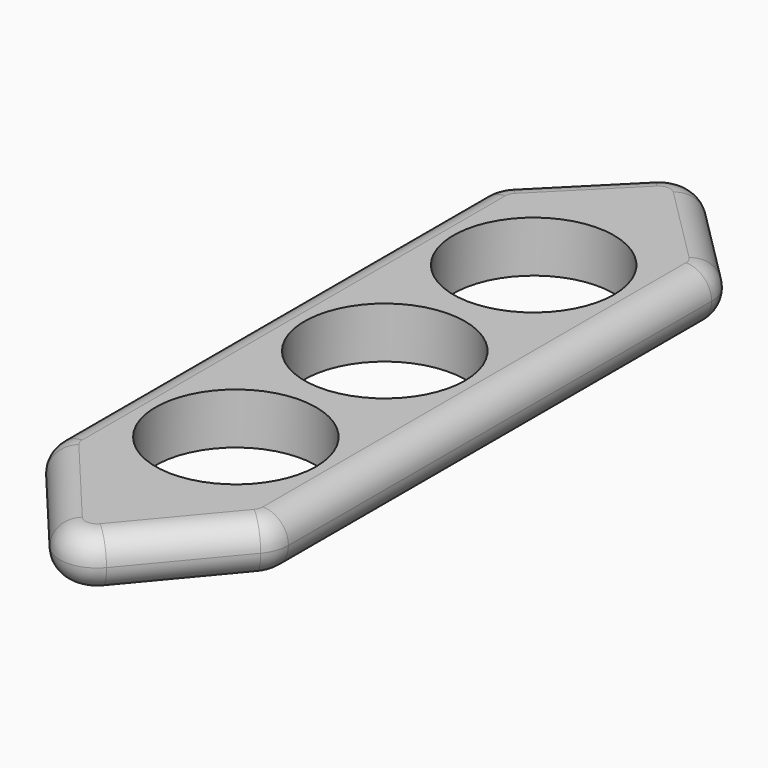
from build123d import *

# Parameters (mm, degrees)
F1_R     = 10.99185
F2_DEPTH = 7
F3_R     = 5.08
F4_R     = 3.49999


# Not quite as in the source:
# - a fillet or chamfer is up to 0.001 mm smaller than in the source, because OpenCascade refuses the exact size


with BuildPart() as f2:
    # F1 (on Top) → F2 (new body)
    with BuildSketch(Plane.XY):
        Polygon((0, 54.0587), (-15.875, 38.1837), (-15.875, -38.1837), (0, -57.15), (15.875, -38.1837), (15.875, 38.1837), align=None)
        with Locations((0, -25.4837)):
            Circle(F1_R, mode=Mode.SUBTRACT)
        Circle(F1_R, mode=Mode.SUBTRACT)
        with Locations((0, 25.4837)):
            Circle(F1_R, mode=Mode.SUBTRACT)
    extrude(amount=F2_DEPTH)

    # F3
    f3_edges = [f2.edges().sort_by_distance(p)[0] for p in [
        (-15.875, -38.1837, 3.5),
        (0, -57.15, 3.5),
        (15.875, -38.1837, 3.5),
        (15.875, 38.1837, 3.5),
        (0, 54.0587, 3.5),
        (-15.875, 38.1837, 3.5),
    ]]
    fillet(f3_edges, radius=F3_R)

    # F4 (radius 3.5 in the source; OpenCascade refuses exactly that, so slightly less here)
    f4_edges = [f2.edges().sort_by_distance(p)[0] for p in [
        (-15.875, -0.129382, 0),
        (15.875, -0.129382, 7),
    ]]
    fillet(f4_edges, radius=F4_R)


solid = f2.part
